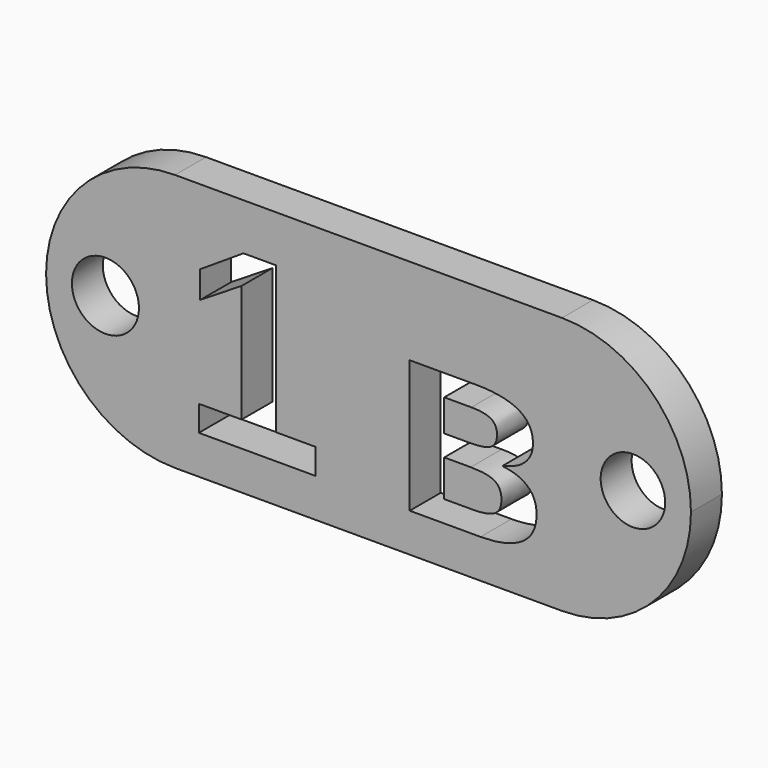
from build123d import *

# Parameters (mm, degrees)
F0_W         = 50
F0_H         = 20
F1_DEPTH     = 3
F2_R         = 2.5
F2_R_2       = 2.6
F2_TEXT_SIZE = 19.4444444444
F3_DEPTH     = 3.001
F4_R         = 9.99999


# Not quite as in the source:
# - a fillet or chamfer is up to 0.001 mm smaller than in the source, because OpenCascade refuses the exact size
# - Text() gives the source's letters only with a copy of the font that has no kerning and outlines rounded to 1/6400 em; it was checked with that copy


with BuildPart() as f1:
    # F0 (on Front) → F1 (new body)
    with BuildSketch(Plane.XZ):
        Rectangle(F0_W, F0_H)
    extrude(amount=F1_DEPTH)

    # F2 (on face) → F3 (cut, through all)
    with BuildSketch(Plane.XZ.offset(3)):
        with Locations((20.5, 0)):
            Circle(F2_R)
        with Locations((-20.4, 0)):
            Circle(F2_R_2)
        with Locations((-14.3782552083, -7)):
            Text('1 в', F2_TEXT_SIZE, font='Arimo', font_style=FontStyle.BOLD, text_align=(TextAlign.LEFT, TextAlign.BOTTOM))
    extrude(amount=-F3_DEPTH, mode=Mode.SUBTRACT)

    # F4 (radius 10 in the source; OpenCascade refuses exactly that, so slightly less here)
    f4_edges = [f1.edges().sort_by_distance(p)[0] for p in [
        (-25, -1.5, 10),
        (-25, -1.5, -10),
        (25, -1.5, 10),
        (25, -1.5, -10),
    ]]
    fillet(f4_edges, radius=F4_R)


solid = f1.part
